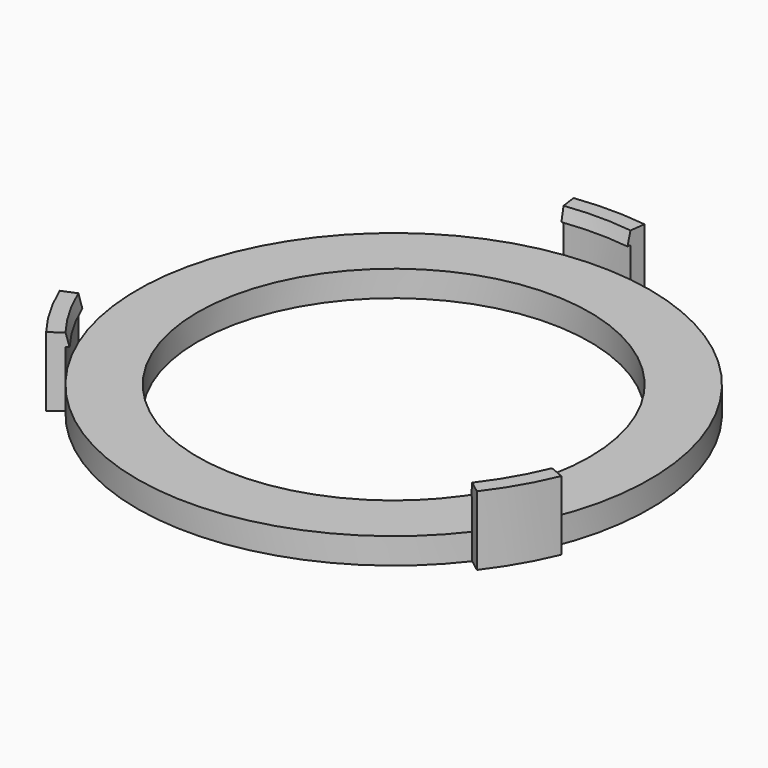
from build123d import *

# Parameters (mm, degrees)
F0_R            = 30.099
F0_R_2          = 23.0124
F1_DEPTH        = 3.048
F3_ANGLE_BACK   = 7.5
F3_ANGLE        = 15
F3_COPIES_COUNT = 3


# Not quite as in the source:
# - a pattern or mirror of a feature is missing from the dataset's text; its kind, count and spacing are read off the source's solid


with BuildPart() as f1:
    # F0 (on Top) → F1 (new body)
    with BuildSketch(Plane.XY):
        Circle(F0_R)
        Circle(F0_R_2, mode=Mode.SUBTRACT)
    extrude(amount=F1_DEPTH)

    # F2 (on Right) → F3 (revolve)
    with BuildSketch(Plane.YZ, mode=Mode.PRIVATE) as f3_sk:
        Polygon((30.099, 6.604), (30.099, 3.048), (30.099, 0), (31.877, 0), (31.877, 8.128), (30.099, 8.128), align=None)
        Polygon((29.718, 6.604), (30.099, 6.604), (30.099, 8.128), align=None)
    f3 = revolve(f3_sk.sketch.rotate(Axis((0, 0, 0), (0, 0, -1)), -F3_ANGLE_BACK), axis=Axis((0, 0, 0), (0, 0, -1)), revolution_arc=F3_ANGLE)

    # F3_copies: F3 ×3 about axis
    f3_copies_axis = Axis((0, 0, 0), (0, 0, 1))
    for i in range(1, F3_COPIES_COUNT):
        add(f3.rotate(f3_copies_axis, i * 360 / F3_COPIES_COUNT))


solid = f1.part
